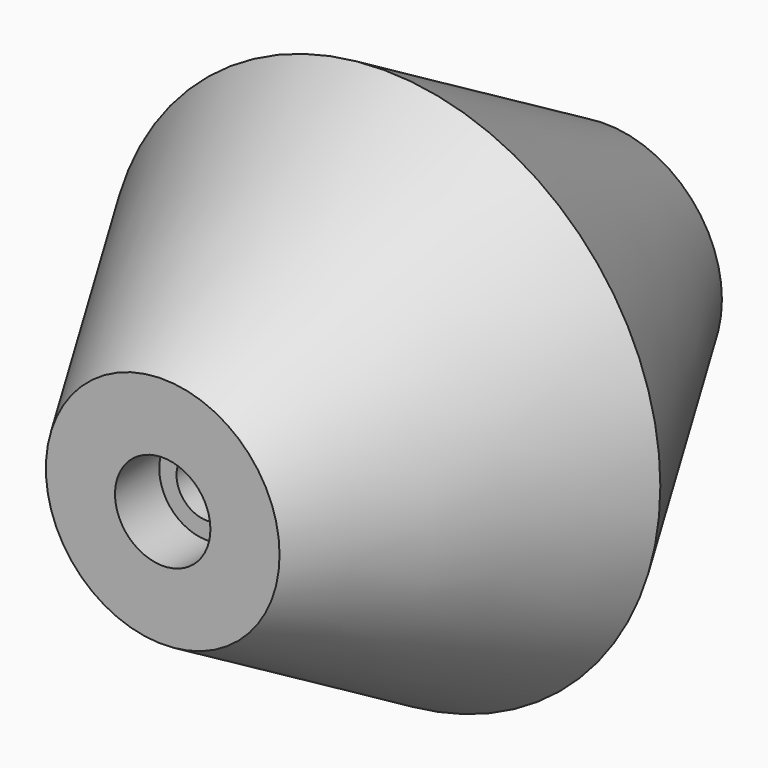
from build123d import *

# Parameters (mm, degrees)
F0_R           = 50
F1_DEPTH       = 50
F1_TAPER       = 30
F3_D           = 11
F3_DEPTH       = 20
F3_CBORE_D     = 17.25
F3_CBORE_DEPTH = 10
F3_TIP         = 3.3047334047


with BuildPart() as f1:
    # F0 (on Front) → F1 (new body, symmetric)
    with BuildSketch(Plane.XZ):
        Circle(F0_R)
    extrude(amount=F1_DEPTH, both=True, taper=F1_TAPER)

    # F3
    with Locations(Plane.XZ.offset(50)):
        with Locations((0, 0)):
            CounterBoreHole(F3_D / 2, F3_CBORE_D / 2, F3_CBORE_DEPTH, depth=F3_DEPTH)
            with Locations((0, 0, -(F3_DEPTH + F3_TIP / 2))):  # 118° drill point
                Cone(0, F3_D / 2, F3_TIP, mode=Mode.SUBTRACT)


solid = f1.part
